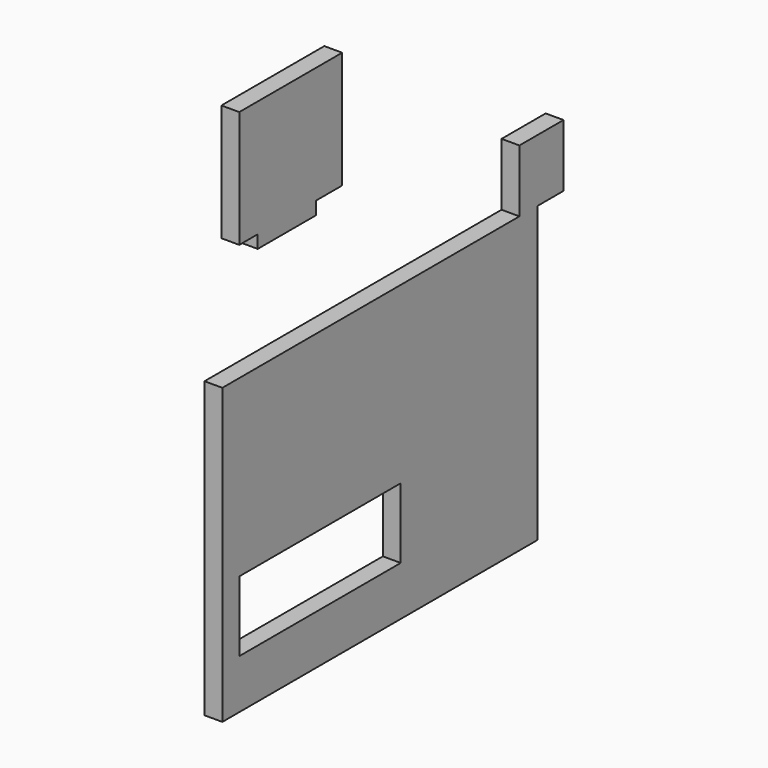
from build123d import *

# Parameters (mm, degrees)
F0_W     = 103.5911440849
F0_H     = 96.5252518654
F0_H_2   = 18.3683950454
F1_DEPTH = 25.4
F0_W_2   = 286.534268409
F0_H_3   = 99.6700823307


with BuildPart() as f1:
    # F0 (on Right) → F1 (new body)
    with BuildSketch(Plane.YZ):
        Polygon((-287.7907156944, 0), (-287.7907156944, 96.5252518654), (-184.1995716095, 96.5252518654), (-184.1995716095, 166.0278588533), (-320.5098807812, 166.0278588533), (-320.5098807812, 0), align=None)
        with Locations((-235.995143652, 48.2626259327)):
            Rectangle(F0_W, F0_H)
        Polygon((-184.1995716095, 166.0278588533), (-184.1995716095, 96.5252518654), (-184.1995716095, 0), (-137.8883123398, 0), (-137.8883123398, 166.0278588533), align=None)
        with Locations((-235.995143652, -9.1841975227)):
            Rectangle(F0_W, F0_H_2)
    extrude(amount=F1_DEPTH)


with BuildPart() as f1b:
    # F0 (on Right) → F1, piece 2 (new body)
    with BuildSketch(Plane.YZ):
        Polygon((255.0225555897, -166.4763987064), (255.0225555897, -77.8435245156), (176.7499446869, -77.8435245156), (176.7499446869, -166.4763987064), (208.9778631926, -166.4763987064), align=None)
        Polygon((208.9778631926, -166.4763987064), (176.7499446869, -166.4763987064), (-350.5717515945, -166.4763987064), (-350.5717515945, -584.1436982155), (208.9778631926, -584.1436982155), align=None)
        with Locations((-177.2427465767, -464.2681926489)):
            Rectangle(F0_W_2, F0_H_3, mode=Mode.SUBTRACT)
    extrude(amount=F1_DEPTH)


solid = Compound([f1.part, f1b.part])
